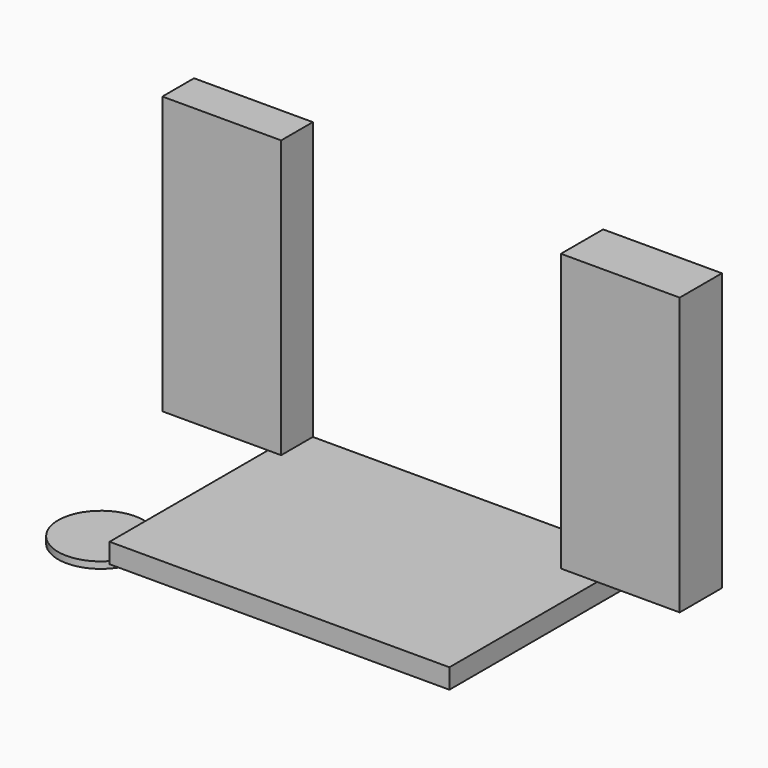
from build123d import *

# Parameters (mm, degrees)
F1_W     = 2616.2
F1_H     = 1828.8
F2_DEPTH = 152.4
F3_W     = 812.8
F3_H     = 304.8
F3_W_2   = 101.6
F4_DEPTH = 2133.6
F3_W_3   = 279.4
F3_H_2   = 406.4
F3_W_4   = 635
F6_R     = 330.2
F7_DEPTH = 50.8


# Not quite as in the source:
# - a variable given as a bare number and used for a length is read in inches; the dataset says mm whatever the document's units were


with BuildPart() as f2:
    # F1 (on Top) → F2 (new body)
    with BuildSketch(Plane.XY):
        Rectangle(F1_W, F1_H)
    extrude(amount=F2_DEPTH)


with BuildPart() as f4:
    # F3 (on face) → F4 (new body)
    with BuildSketch(Plane.XY.offset(152.4)):
        with Locations((-1714.5, 762)):
            Rectangle(F3_W, F3_H)
        with Locations((-1257.3, 762)):
            Rectangle(F3_W_2, F3_H)
    extrude(amount=F4_DEPTH)


with BuildPart() as f4b:
    # F3 (on face) → F4, piece 2 (new body)
    with BuildSketch(Plane.XY.offset(152.4)):
        with Locations((1168.4, 711.2)):
            Rectangle(F3_W_3, F3_H_2)
        with Locations((1625.6, 711.2)):
            Rectangle(F3_W_4, F3_H_2)
    extrude(amount=F4_DEPTH)


with BuildPart() as f7:
    # F6 (on offset) → F7 (new body)
    with BuildSketch(Plane.XY.offset(-50.8)):
        with Locations((-1638.3, -584.2)):
            Circle(F6_R)
    extrude(amount=-F7_DEPTH)


solid = Compound([f2.part, f4.part, f4b.part, f7.part])
